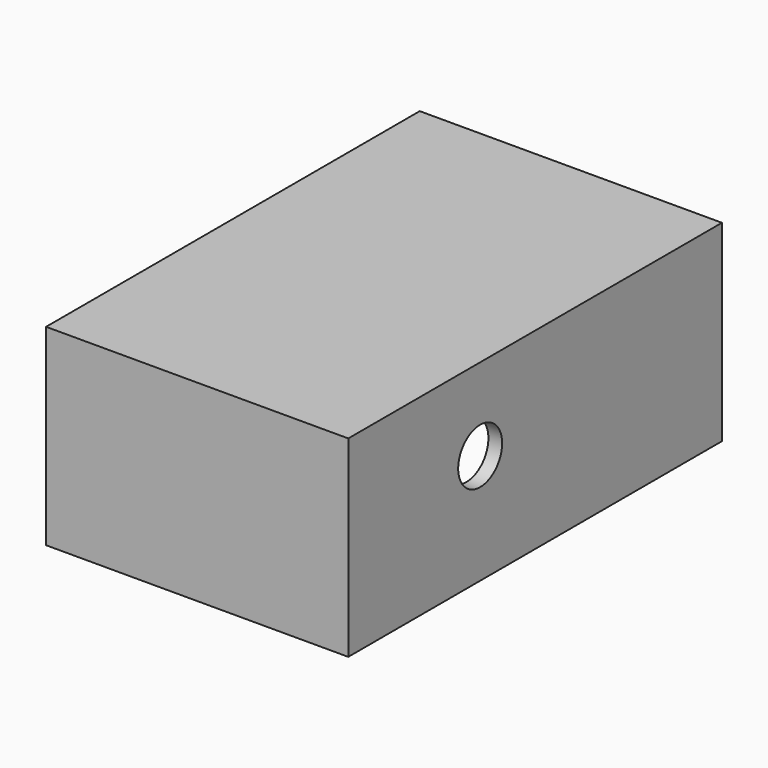
from build123d import *

# Parameters (mm, degrees)
F0_W     = 55
F0_H     = 85
F1_DEPTH = 35
F3_T     = -2.5
F4_R     = 5
F5_DEPTH = 25


# Not quite as in the source:
# - the program builds the solid bodies; features that only make, move or delete a surface that nothing else refers to are left out


with BuildPart() as f1:
    # F0 (on Top) → F1 (new body)
    with BuildSketch(Plane.XY):
        with Locations((-28.1140384175, 11.1121237278)):
            Rectangle(F0_W, F0_H)
    extrude(amount=F1_DEPTH)

    # F3
    f3_openings = [f1.faces().sort_by_distance(p)[0] for p in [
        (-28.114038, 11.112124, 0),
    ]]
    offset(amount=F3_T, openings=f3_openings)

    # F4 (on face) → F5 (cut)
    with BuildSketch(Plane.YZ.offset(-0.6140384175)):
        with Locations((-1.3878762722, 20)):
            Circle(F4_R)
    extrude(amount=-F5_DEPTH, mode=Mode.SUBTRACT)


solid = f1.part
